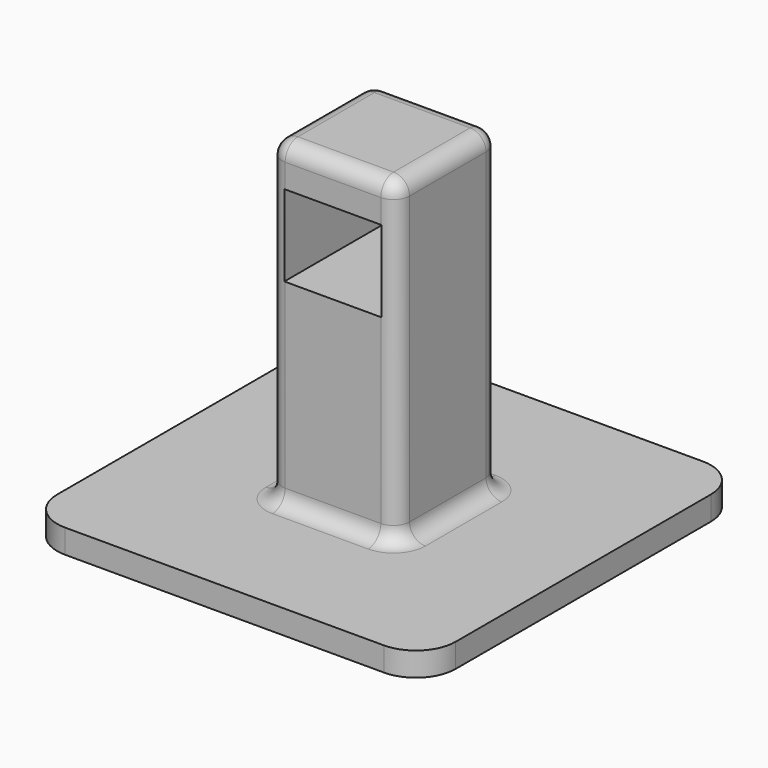
from build123d import *

# Parameters (mm, degrees)
F0_W         = 50
F0_H         = 50
F1_DEPTH     = 3
F2_W         = 16
F2_H         = 16
F3_DEPTH     = 40
F4_W         = 12.2
F4_H         = 10.2
F5_DEPTH     = 16
F6_T1_DEPTH  = 12
F6_T3_DEPTH  = 12
F6_T5_DEPTH  = 38
F6_S9_W      = 2
F6_S9_H      = 2
F6_T10_DEPTH = 2
F6_S15_W     = 2
F6_S15_H     = 2
F6_T16_DEPTH = 2
F6_S21_W     = 2
F6_S21_H     = 2
F6_T22_DEPTH = 2
F6_S27_W     = 2
F6_S27_H     = 2
F6_T28_DEPTH = 2
F6_T31_DEPTH = 12
F6_T33_DEPTH = 12
F6_T36_ANGLE = 90
F6_T38_ANGLE = 90
F6_T40_ANGLE = 90
F6_T42_ANGLE = 90
F7_R         = 5


# Not quite as in the source:
# - a fillet or chamfer that OpenCascade refuses, or shapes differently, is made with other operations: its cross-section is extruded or revolved along the edge and cut away or added


with BuildPart() as f1:
    # F0 (on Top) → F1 (new body)
    with BuildSketch(Plane.XY):
        with Locations((25, 25)):
            Rectangle(F0_W, F0_H)
    extrude(amount=F1_DEPTH)

    # F2 (on face) → F3 (join)
    with BuildSketch(Plane.XY.offset(3)):
        with Locations((25, 25)):
            Rectangle(F2_W, F2_H)
    extrude(amount=F3_DEPTH)

    # F4 (on face) → F5 (cut)
    with BuildSketch(Plane.XZ.offset(-17)):
        with Locations((25, 32.9)):
            Rectangle(F4_W, F4_H)
    extrude(amount=-F5_DEPTH, mode=Mode.SUBTRACT)

    # F6: fillet of radius 2 on 12 edges, made by hand

    # F6_s2 → F6_t1 (cut)
    with BuildSketch(Plane.YZ.offset(19)):
        with BuildLine():
            ThreePointArc((17, 41), (17.5857864376, 42.4142135624), (19, 43))
            Line((19, 43), (17, 43))
            Line((17, 43), (17, 41))
        make_face()
        with BuildLine():
            ThreePointArc((33, 41), (32.4142135624, 42.4142135624), (31, 43))
            Line((31, 43), (33, 43))
            Line((33, 43), (33, 41))
        make_face()
    extrude(amount=F6_T1_DEPTH, mode=Mode.SUBTRACT)

    # F6_s4 → F6_t3 (cut)
    with BuildSketch(Plane.XZ.offset(-31)):
        with BuildLine():
            ThreePointArc((33, 41), (32.4142135624, 42.4142135624), (31, 43))
            Line((31, 43), (33, 43))
            Line((33, 43), (33, 41))
        make_face()
        with BuildLine():
            ThreePointArc((17, 41), (17.5857864376, 42.4142135624), (19, 43))
            Line((19, 43), (17, 43))
            Line((17, 43), (17, 41))
        make_face()
    extrude(amount=F6_T3_DEPTH, mode=Mode.SUBTRACT)

    # F6_s6 → F6_t5 (cut)
    with BuildSketch(Plane.XY.offset(3)):
        with BuildLine():
            ThreePointArc((31, 17), (32.4142135624, 17.5857864376), (33, 19))
            Line((33, 19), (33, 17))
            Line((33, 17), (31, 17))
        make_face()
        with BuildLine():
            ThreePointArc((31, 33), (32.4142135624, 32.4142135624), (33, 31))
            Line((33, 31), (33, 33))
            Line((33, 33), (31, 33))
        make_face()
        with BuildLine():
            ThreePointArc((17, 19), (17.5857864376, 17.5857864376), (19, 17))
            Line((19, 17), (17, 17))
            Line((17, 17), (17, 19))
        make_face()
        with BuildLine():
            ThreePointArc((19, 33), (17.5857864376, 32.4142135624), (17, 31))
            Line((17, 31), (17, 33))
            Line((17, 33), (19, 33))
        make_face()
    extrude(amount=F6_T5_DEPTH, mode=Mode.SUBTRACT)


with BuildPart() as f6_tool8:
    # F6_s9 → F6_t10 (new body)
    with BuildSketch(Plane.XZ.offset(-19)):
        with Locations((18, 42)):
            Rectangle(F6_S9_W, F6_S9_H)
    extrude(amount=F6_T10_DEPTH)

    # F6_s11 → F6_t12 (revolve, cut)
    with BuildSketch(Plane(origin=(19, 19, 41), x_dir=(0.7071067812, 0, -0.7071067812), z_dir=(-0.7071067812, 0, -0.7071067812))):
        with BuildLine():
            ThreePointArc((0, -2), (2, 0), (0, 2))
            Line((0, 2), (0, -2))
        make_face()
    revolve(axis=Axis((19, 19, 41), (0, -1, 0)), mode=Mode.SUBTRACT)


with BuildPart() as f1_1:
    add(f1.part)

    # F6_t7: cut F6_tool8
    add(f6_tool8.part, mode=Mode.SUBTRACT)


with BuildPart() as f6_tool14:
    # F6_s15 → F6_t16 (new body)
    with BuildSketch(Plane.XZ.offset(-19)):
        with Locations((32, 42)):
            Rectangle(F6_S15_W, F6_S15_H)
    extrude(amount=F6_T16_DEPTH)

    # F6_s17 → F6_t18 (revolve, cut)
    with BuildSketch(Plane(origin=(31, 19, 41), x_dir=(-0.7071067812, 0, -0.7071067812), z_dir=(-0.7071067812, 0, 0.7071067812))):
        with BuildLine():
            ThreePointArc((0, -2), (2, 0), (0, 2))
            Line((0, 2), (0, -2))
        make_face()
    revolve(axis=Axis((31, 19, 41), (0, -1, 0)), mode=Mode.SUBTRACT)


with BuildPart() as f1_2:
    add(f1_1.part)

    # F6_t13: cut F6_tool14
    add(f6_tool14.part, mode=Mode.SUBTRACT)


with BuildPart() as f6_tool20:
    # F6_s21 → F6_t22 (new body)
    with BuildSketch(Plane.YZ.offset(31)):
        with Locations((32, 42)):
            Rectangle(F6_S21_W, F6_S21_H)
    extrude(amount=F6_T22_DEPTH)

    # F6_s23 → F6_t24 (revolve, cut)
    with BuildSketch(Plane(origin=(31, 31, 41), x_dir=(0, -0.7071067812, -0.7071067812), z_dir=(0, -0.7071067812, 0.7071067812))):
        with BuildLine():
            ThreePointArc((0, -2), (2, 0), (0, 2))
            Line((0, 2), (0, -2))
        make_face()
    revolve(axis=Axis((31, 31, 41), (1, 0, 0)), mode=Mode.SUBTRACT)


with BuildPart() as f1_3:
    add(f1_2.part)

    # F6_t19: cut F6_tool20
    add(f6_tool20.part, mode=Mode.SUBTRACT)


with BuildPart() as f6_tool26:
    # F6_s27 → F6_t28 (new body)
    with BuildSketch(Plane.XY.offset(41)):
        with Locations((18, 32)):
            Rectangle(F6_S27_W, F6_S27_H)
    extrude(amount=F6_T28_DEPTH)

    # F6_s29 → F6_t30 (revolve, cut)
    with BuildSketch(Plane(origin=(19, 31, 41), x_dir=(0.7071067812, -0.7071067812, 0), z_dir=(-0.7071067812, -0.7071067812, 0))):
        with BuildLine():
            ThreePointArc((0, -2), (2, 0), (0, 2))
            Line((0, 2), (0, -2))
        make_face()
    revolve(axis=Axis((19, 31, 41), (0, 0, 1)), mode=Mode.SUBTRACT)


with BuildPart() as f1_4:
    add(f1_3.part)

    # F6_t25: cut F6_tool26
    add(f6_tool26.part, mode=Mode.SUBTRACT)

    # F6_s32 → F6_t31 (join)
    with BuildSketch(Plane.YZ.offset(19)):
        with BuildLine():
            ThreePointArc((15, 3), (16.4142135624, 3.5857864376), (17, 5))
            Line((17, 5), (17, 3))
            Line((17, 3), (15, 3))
        make_face()
        with BuildLine():
            ThreePointArc((35, 3), (33.5857864376, 3.5857864376), (33, 5))
            Line((33, 5), (33, 3))
            Line((33, 3), (35, 3))
        make_face()
    extrude(amount=F6_T31_DEPTH)

    # F6_s34 → F6_t33 (join)
    with BuildSketch(Plane.XZ.offset(-31)):
        with BuildLine():
            ThreePointArc((35, 3), (33.5857864376, 3.5857864376), (33, 5))
            Line((33, 5), (33, 3))
            Line((33, 3), (35, 3))
        make_face()
        with BuildLine():
            ThreePointArc((15, 3), (16.4142135624, 3.5857864376), (17, 5))
            Line((17, 5), (17, 3))
            Line((17, 3), (15, 3))
        make_face()
    extrude(amount=F6_T33_DEPTH)

    # F6_s35 → F6_t36 (revolve)
    with BuildSketch(Plane.YZ.offset(31)):
        with BuildLine():
            ThreePointArc((35, 3), (33.5857864376, 3.5857864376), (33, 5))
            Line((33, 5), (33, 3))
            Line((33, 3), (35, 3))
        make_face()
    revolve(axis=Axis((31, 31, 3), (0, 0, -1)), revolution_arc=F6_T36_ANGLE)

    # F6_s37 → F6_t38 (revolve)
    with BuildSketch(Plane.YZ.offset(19)):
        with BuildLine():
            ThreePointArc((35, 3), (33.5857864376, 3.5857864376), (33, 5))
            Line((33, 5), (33, 3))
            Line((33, 3), (35, 3))
        make_face()
    revolve(axis=Axis((19, 31, 3), (0, 0, 1)), revolution_arc=F6_T38_ANGLE)

    # F6_s39 → F6_t40 (revolve)
    with BuildSketch(Plane.XZ.offset(-19)):
        with BuildLine():
            ThreePointArc((15, 3), (16.4142135624, 3.5857864376), (17, 5))
            Line((17, 5), (17, 3))
            Line((17, 3), (15, 3))
        make_face()
    revolve(axis=Axis((19, 19, 3), (0, 0, 1)), revolution_arc=F6_T40_ANGLE)

    # F6_s41 → F6_t42 (revolve)
    with BuildSketch(Plane.YZ.offset(31)):
        with BuildLine():
            ThreePointArc((15, 3), (16.4142135624, 3.5857864376), (17, 5))
            Line((17, 5), (17, 3))
            Line((17, 3), (15, 3))
        make_face()
    revolve(axis=Axis((31, 19, 3), (0, 0, 1)), revolution_arc=F6_T42_ANGLE)

    # F7
    f7_edges = [f1_4.edges().sort_by_distance(p)[0] for p in [
        (0, 0, 1.5),
        (50, 0, 1.5),
        (0, 50, 1.5),
        (50, 50, 1.5),
    ]]
    fillet(f7_edges, radius=F7_R)


solid = f1_4.part
